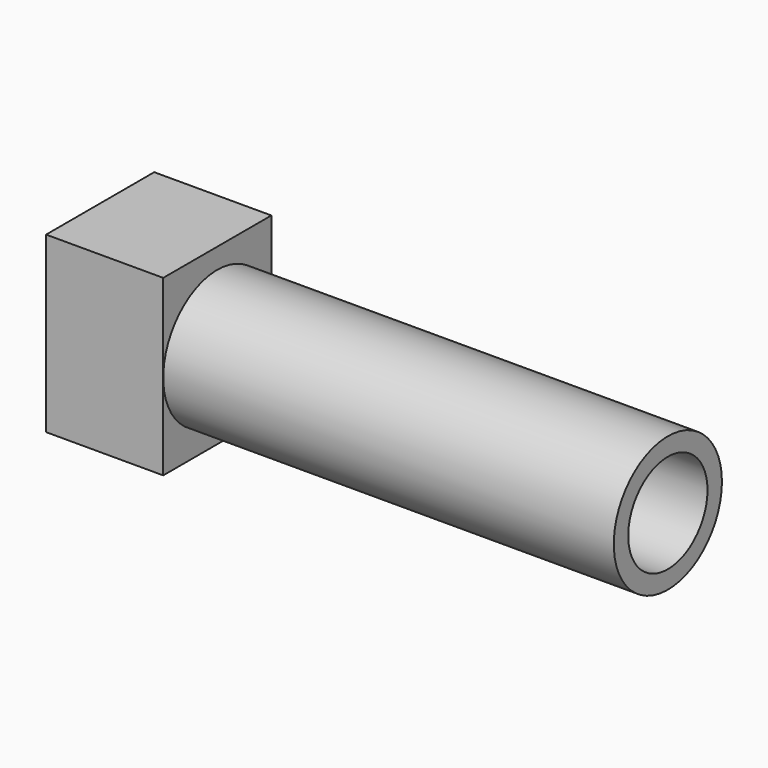
from build123d import *

# Parameters (mm, degrees)
F0_R     = 19.05
F0_R_2   = 13.97
F1_DEPTH = 127
F2_W     = 38.0999972801
F2_H     = 49.0219972801
F2_W_2   = 30.988
F2_H_2   = 41.91
F3_DEPTH = 33.02
F8_W     = 30.988
F8_H     = 41.91
F9_DEPTH = 32.004


# Not quite as in the source:
# - the program builds the solid bodies; features that only make, move or delete a surface that nothing else refers to are left out


with BuildPart() as f1:
    # F0 (on Right) → F1 (new body)
    with BuildSketch(Plane.YZ):
        Circle(F0_R)
        Circle(F0_R_2, mode=Mode.SUBTRACT)
    extrude(amount=F1_DEPTH)


with BuildPart() as f3:
    # F2 (on Right) → F3 (new body)
    with BuildSketch(Plane.YZ):
        with Locations((-0.0063063291, 0.2760496718)):
            Rectangle(F2_W, F2_H)
        with Locations((-0.0063063291, 0.2760496718)):
            Rectangle(F2_W_2, F2_H_2, mode=Mode.SUBTRACT)
        with Locations((-0.0063063291, 0.2760496718)):
            Rectangle(F2_W_2, F2_H_2)
    extrude(amount=-F3_DEPTH)

    # F8 (on face) → F9 (cut)
    with BuildSketch(Plane(origin=(-33.02, 0, 0), x_dir=(0, -1, 0), z_dir=(-1, 0, 0))):
        with Locations((0.0792781701, 0.2760499603)):
            Rectangle(F8_W, F8_H)
    extrude(amount=-F9_DEPTH, mode=Mode.SUBTRACT)


solid = Compound([f1.part, f3.part])
